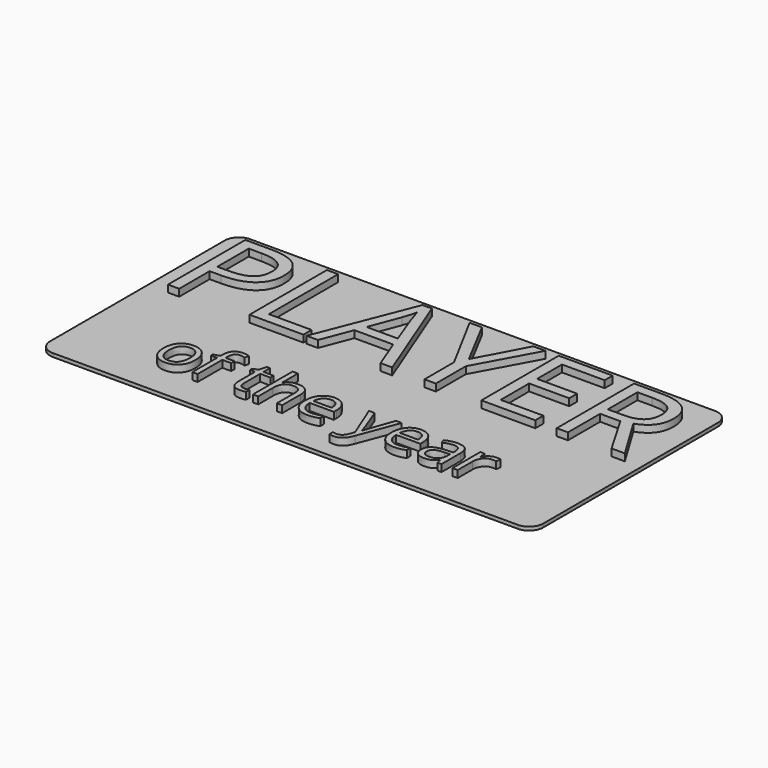
from build123d import *

# Parameters (mm, degrees)
F0_W           = 70
F0_H           = 35
F1_DEPTH       = 0.5
F2_R           = 2
F3_TEXT_SIZE   = 9.2645278972
F3_TEXT_SIZE_2 = 19.2241774392
F4_DEPTH       = 1


# Not quite as in the source:
# - Text() gives the source's letters only with a copy of the font that has no kerning and outlines rounded to 1/6400 em; it was checked with that copy


with BuildPart() as f1:
    # F0 (on Top) → F1 (new body)
    with BuildSketch(Plane.XY):
        with Locations((14.7194565833, -21.0120362043)):
            Rectangle(F0_W, F0_H)
    extrude(amount=-F1_DEPTH)

    # F2
    f2_edges = [f1.edges().sort_by_distance(p)[0] for p in [
        (49.719457, -38.512036, -0.25),
        (-20.280543, -38.512036, -0.25),
        (-20.280543, -3.512036, -0.25),
        (49.719457, -3.512036, -0.25),
    ]]
    fillet(f2_edges, radius=F2_R)


with BuildPart() as f4:
    # F3 (on Top) → F4 (new body)
    with BuildSketch(Plane.XY):
        with Locations((-8.7682930099, -33.9198224057)):
            Text('of the year', F3_TEXT_SIZE, font='Open Sans', text_align=(TextAlign.LEFT, TextAlign.BOTTOM))
        with Locations((-19.2690128461, -19.2111785625)):
            Text('PLAYER', F3_TEXT_SIZE_2, font='Open Sans', text_align=(TextAlign.LEFT, TextAlign.BOTTOM))
    extrude(amount=F4_DEPTH)


solid = Compound([f1.part, f4.part])
